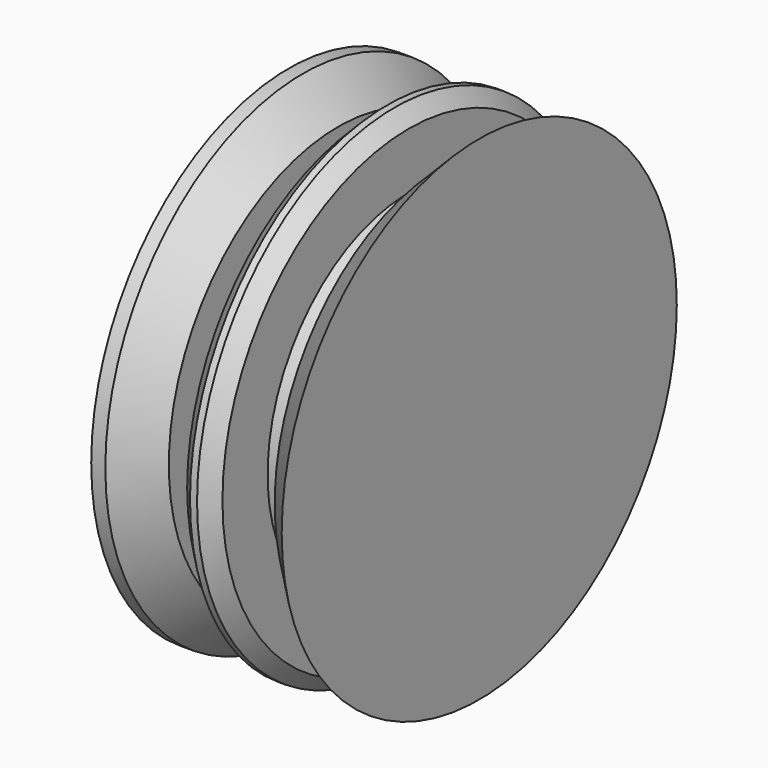
from build123d import *

# Parameters (mm, degrees)
F0_R      = 35
F1_DEPTH  = 7
F2_R      = 25
F3_DEPTH  = 5
F5_R      = 35
F6_DEPTH  = 5
F7_R      = 25
F8_DEPTH  = 5
F9_R      = 35
F10_DEPTH = 5
F11_SIZE  = 4.99999
F12_SIZE  = 2


# Not quite as in the source:
# - a fillet or chamfer is up to 0.001 mm smaller than in the source, because OpenCascade refuses the exact size


with BuildPart() as f1:
    # F0 (on Right) → F1 (new body)
    with BuildSketch(Plane.YZ):
        Circle(F0_R)
    extrude(amount=F1_DEPTH)

    # F2 (on face) → F3 (join)
    with BuildSketch(Plane.YZ.offset(7)):
        Circle(F2_R)
    extrude(amount=F3_DEPTH)

    # F5 (on face) → F6 (join)
    with BuildSketch(Plane.YZ.offset(12)):
        Circle(F5_R)
    extrude(amount=F6_DEPTH)

    # F7 (on face) → F8 (join)
    with BuildSketch(Plane.YZ.offset(17)):
        Circle(F7_R)
    extrude(amount=F8_DEPTH)

    # F9 (on face) → F10 (join)
    with BuildSketch(Plane.YZ.offset(22)):
        Circle(F9_R)
    extrude(amount=F10_DEPTH)

    # F11 (size 5 in the source; OpenCascade refuses exactly that, so slightly less here)
    f11_edges = [f1.edges().sort_by_distance(p)[0] for p in [
        (7, -35, 0),
        (22, -35, 0),
    ]]
    chamfer(f11_edges, length=F11_SIZE)

    # F12
    f12_edges = [f1.edges().sort_by_distance(p)[0] for p in [
        (12, -35, 0),
        (17, -35, 0),
    ]]
    chamfer(f12_edges, length=F12_SIZE)


solid = f1.part
